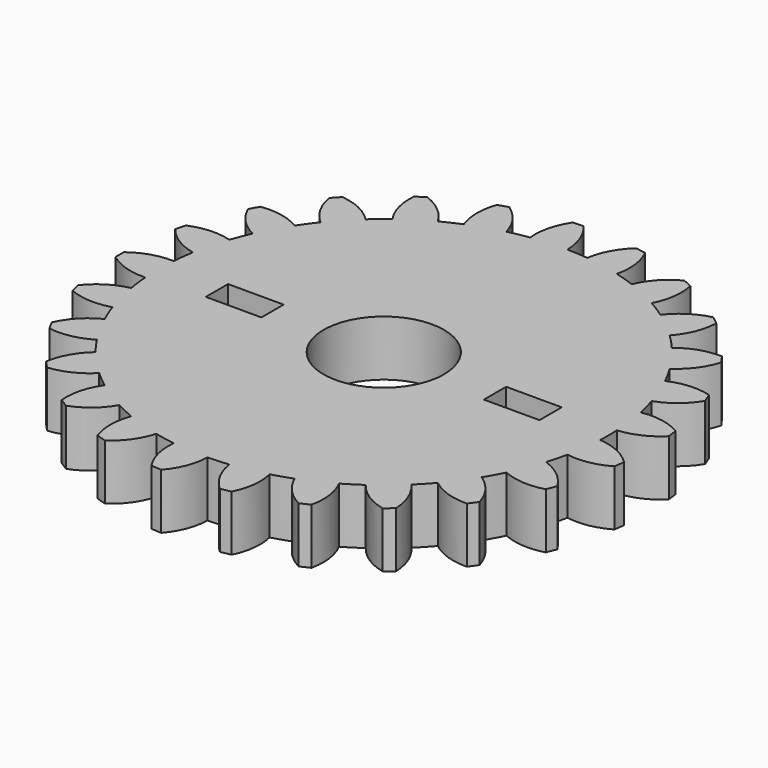
from build123d import *

# Parameters (mm, degrees)
F1_W     = 6
F1_H     = 3
F1_R     = 6.5
F2_DEPTH = 6


# Not quite as in the source:
# - a feature names something its author has since deleted; it is built from what else it names


with BuildPart() as f2:
    # F1 (on Top) → F2 (new body)
    with BuildSketch(Plane.XY):
        with BuildLine():
            ThreePointArc((2.6492001042, 24.1328040773), (1.5244142797, 24.2298711291), (0.3963319999, 24.2745425245))
            ThreePointArc((0.3963319999, 24.2745425245), (-0.0481990645, 26.5171542751), (-1.2314510555, 28.4733828039))
            Line((-1.2314510555, 28.4733828039), (-2.3469204412, 28.4032034187))
            ThreePointArc((-2.3469204412, 28.4032034187), (-3.2756616898, 26.314099538), (-3.4356137115, 24.0334569351))
            ThreePointArc((-3.4356137115, 24.0334569351), (-4.5492019152, 23.8477515871), (-5.6529527401, 23.6104768936))
            ThreePointArc((-5.6529527401, 23.6104768936), (-6.6412329068, 25.672082492), (-8.2738051128, 27.2725897002))
            Line((-8.2738051128, 27.2725897002), (-9.3367770732, 26.9272091737))
            ThreePointArc((-9.3367770732, 26.9272091737), (-9.7168011992, 24.6727697767), (-9.3045552825, 22.4239993048))
            ThreePointArc((-9.3045552825, 22.4239993048), (-10.336975023, 21.9671901071), (-11.3470416693, 21.4628781663))
            ThreePointArc((-11.3470416693, 21.4628781663), (-12.8169736609, 23.2139393506), (-14.796285566, 24.358159484))
            Line((-14.796285566, 24.358159484), (-15.7399696634, 23.7592793451))
            ThreePointArc((-15.7399696634, 23.7592793451), (-15.5473983534, 21.4811591503), (-14.5888574253, 19.4055593285))
            ThreePointArc((-14.5888574253, 19.4055593285), (-15.4752379733, 18.7063492829), (-16.3281542389, 17.9666878688))
            ThreePointArc((-16.3281542389, 17.9666878688), (-18.1873768224, 19.297179025), (-20.3890609801, 19.9132165245))
            Line((-20.3890609801, 19.9132165245), (-21.1541620721, 19.0984666146))
            ThreePointArc((-21.1541620721, 19.0984666146), (-20.4010952897, 16.9398082923), (-18.9564880021, 15.1677966909))
            ThreePointArc((-18.9564880021, 15.1677966909), (-19.6411348079, 14.2701197362), (-20.283308827, 13.3415844957))
            ThreePointArc((-20.283308827, 13.3415844957), (-22.4150002096, 14.1679059711), (-24.7007167071, 14.217052935))
            Line((-24.7007167071, 14.217052935), (-25.2391606782, 13.2376269875))
            ThreePointArc((-25.2391606782, 13.2376269875), (-23.972916379, 11.334066979), (-22.1330127205, 9.9769856039))
            ThreePointArc((-22.1330127205, 9.9769856039), (-22.5729069074, 8.9372460846), (-22.9639885246, 7.8781803018))
            ThreePointArc((-22.9639885246, 7.8781803018), (-25.234206697, 8.1484112791), (-27.4603355605, 7.6275796229))
            Line((-27.4603355605, 7.6275796229), (-27.7382899958, 6.5450185722))
            ThreePointArc((-27.7382899958, 6.5450185722), (-26.038430966, 5.0161645537), (-23.9188388502, 4.1592838187))
            ThreePointArc((-23.9188388502, 4.1592838187), (-24.0863402486, 3.0428123926), (-24.2017563676, 1.9197610656))
            ThreePointArc((-24.2017563676, 1.9197610656), (-26.4678551727, 1.6169219388), (-28.4945205386, 0.5588374309))
            Line((-28.4945205386, 0.5588374309), (-28.4945205386, -0.5588374309))
            ThreePointArc((-28.4945205386, -0.5588374309), (-26.4678551727, -1.6169219388), (-24.2017563676, -1.9197610656))
            ThreePointArc((-24.2017563676, -1.9197610656), (-24.0863402486, -3.0428123926), (-23.9188388502, -4.1592838187))
            ThreePointArc((-23.9188388502, -4.1592838187), (-26.038430966, -5.0161645537), (-27.7382899958, -6.5450185722))
            Line((-27.7382899958, -6.5450185722), (-27.4603355605, -7.6275796229))
            ThreePointArc((-27.4603355605, -7.6275796229), (-25.234206697, -8.1484112791), (-22.9639885246, -7.8781803018))
            ThreePointArc((-22.9639885246, -7.8781803018), (-22.5729069074, -8.9372460846), (-22.1330127205, -9.9769856039))
            ThreePointArc((-22.1330127205, -9.9769856039), (-23.972916379, -11.334066979), (-25.2391606782, -13.2376269875))
            Line((-25.2391606782, -13.2376269875), (-24.7007167071, -14.217052935))
            ThreePointArc((-24.7007167071, -14.217052935), (-22.4150002096, -14.1679059711), (-20.283308827, -13.3415844957))
            ThreePointArc((-20.283308827, -13.3415844957), (-19.6411348079, -14.2701197362), (-18.9564880021, -15.1677966909))
            ThreePointArc((-18.9564880021, -15.1677966909), (-20.4010952897, -16.9398082923), (-21.1541620721, -19.0984666146))
            Line((-21.1541620721, -19.0984666146), (-20.3890609801, -19.9132165245))
            ThreePointArc((-20.3890609801, -19.9132165245), (-18.1873768224, -19.297179025), (-16.3281542389, -17.9666878688))
            ThreePointArc((-16.3281542389, -17.9666878688), (-15.4752379733, -18.7063492829), (-14.5888574253, -19.4055593285))
            ThreePointArc((-14.5888574253, -19.4055593285), (-15.5473983534, -21.4811591503), (-15.7399696634, -23.7592793451))
            Line((-15.7399696634, -23.7592793451), (-14.796285566, -24.358159484))
            ThreePointArc((-14.796285566, -24.358159484), (-12.8169736609, -23.2139393506), (-11.3470416693, -21.4628781663))
            ThreePointArc((-11.3470416693, -21.4628781663), (-10.336975023, -21.9671901071), (-9.3045552825, -22.4239993048))
            ThreePointArc((-9.3045552825, -22.4239993048), (-9.7168011992, -24.6727697767), (-9.3367770732, -26.9272091737))
            Line((-9.3367770732, -26.9272091737), (-8.2738051128, -27.2725897002))
            ThreePointArc((-8.2738051128, -27.2725897002), (-6.6412329068, -25.672082492), (-5.6529527401, -23.6104768936))
            ThreePointArc((-5.6529527401, -23.6104768936), (-4.5492019152, -23.8477515871), (-3.4356137115, -24.0334569351))
            ThreePointArc((-3.4356137115, -24.0334569351), (-3.2756616898, -26.314099538), (-2.3469204412, -28.4032034187))
            Line((-2.3469204412, -28.4032034187), (-1.2314510555, -28.4733828039))
            ThreePointArc((-1.2314510555, -28.4733828039), (-0.0481990645, -26.5171542751), (0.3963319999, -24.2745425245))
            ThreePointArc((0.3963319999, -24.2745425245), (1.5244142797, -24.2298711291), (2.6492001042, -24.1328040773))
            ThreePointArc((2.6492001042, -24.1328040773), (3.3712996907, -26.3020176488), (4.7904018334, -28.0945199331))
            Line((4.7904018334, -28.0945199331), (5.8882796006, -27.8850885483))
            ThreePointArc((5.8882796006, -27.8850885483), (6.5478633024, -25.6960557318), (6.4207137427, -23.413349373))
            ThreePointArc((6.4207137427, -23.413349373), (7.502245919, -23.0895387567), (8.5675549344, -22.7157983851))
            ThreePointArc((8.5675549344, -22.7157983851), (9.8064299128, -24.6372832586), (11.626725543, -26.0205544358))
            Line((11.626725543, -26.0205544358), (12.6380279938, -25.544671625))
            ThreePointArc((12.6380279938, -25.544671625), (12.7324993366, -23.2603795034), (12.0416584273, -21.0810093721))
            ThreePointArc((12.0416584273, -21.0810093721), (13.0086838559, -20.4984057469), (13.9475787787, -19.8714755375))
            ThreePointArc((13.9475787787, -19.8714755375), (15.6253860779, -21.4244977518), (17.7324993267, -22.3116218064))
            Line((17.7324993267, -22.3116218064), (18.5936826087, -21.5991890368))
            ThreePointArc((18.5936826087, -21.5991890368), (18.1171056106, -19.3631680851), (16.9059814268, -17.4240720219))
            ThreePointArc((16.9059814268, -17.4240720219), (17.6977383435, -16.6192825162), (18.4512249528, -15.7785547997))
            ThreePointArc((18.4512249528, -15.7785547997), (20.4625417697, -16.8655322574), (22.724074962, -17.2007679224))
            Line((22.724074962, -17.2007679224), (23.3810277626, -16.2965499651))
            ThreePointArc((23.3810277626, -16.2965499651), (22.3633475091, -14.2492976033), (20.7080394374, -12.6723161452))
            ThreePointArc((20.7080394374, -12.6723161452), (21.2747788433, -11.6959086435), (21.7955128043, -10.6942094344))
            ThreePointArc((21.7955128043, -10.6942094344), (24.0139607061, -11.2468433441), (26.2878133942, -11.0091265299))
            Line((26.2878133942, -11.0091265299), (26.6992569527, -9.9699387246))
            ThreePointArc((26.6992569527, -9.9699387246), (25.2044180369, -8.2400913478), (23.2089351714, -7.1243120397))
            ThreePointArc((23.2089351714, -7.1243120397), (23.5150467452, -6.0376378162), (23.7703084279, -4.9379075597))
            ThreePointArc((23.7703084279, -4.9379075597), (26.0564941741, -4.9214739006), (28.199791831, -4.1257412288))
            Line((28.199791831, -4.1257412288), (28.3398736355, -3.0168795672))
            ThreePointArc((28.3398736355, -3.0168795672), (26.4618022841, -1.713129848), (24.251528152, -1.1286612073))
            ThreePointArc((24.251528152, -1.1286612073), (24.2777777778, 0), (24.251528152, 1.1286612073))
            ThreePointArc((24.251528152, 1.1286612073), (26.4618022841, 1.713129848), (28.3398736355, 3.0168795672))
            Line((28.3398736355, 3.0168795672), (28.199791831, 4.1257412288))
            ThreePointArc((28.199791831, 4.1257412288), (26.0564941741, 4.9214739006), (23.7703084279, 4.9379075597))
            ThreePointArc((23.7703084279, 4.9379075597), (23.5150467452, 6.0376378162), (23.2089351714, 7.1243120397))
            ThreePointArc((23.2089351714, 7.1243120397), (25.2044180369, 8.2400913478), (26.6992569527, 9.9699387246))
            Line((26.6992569527, 9.9699387246), (26.2878133942, 11.0091265299))
            ThreePointArc((26.2878133942, 11.0091265299), (24.0139607061, 11.2468433441), (21.7955128043, 10.6942094344))
            ThreePointArc((21.7955128043, 10.6942094344), (21.2747788433, 11.6959086435), (20.7080394374, 12.6723161452))
            ThreePointArc((20.7080394374, 12.6723161452), (22.3633475091, 14.2492976033), (23.3810277626, 16.2965499651))
            Line((23.3810277626, 16.2965499651), (22.724074962, 17.2007679224))
            ThreePointArc((22.724074962, 17.2007679224), (20.4625417697, 16.8655322574), (18.4512249528, 15.7785547997))
            ThreePointArc((18.4512249528, 15.7785547997), (17.6977383435, 16.6192825162), (16.9059814268, 17.4240720219))
            ThreePointArc((16.9059814268, 17.4240720219), (18.1171056106, 19.3631680851), (18.5936826087, 21.5991890368))
            Line((18.5936826087, 21.5991890368), (17.7324993267, 22.3116218064))
            ThreePointArc((17.7324993267, 22.3116218064), (15.6253860779, 21.4244977518), (13.9475787787, 19.8714755375))
            ThreePointArc((13.9475787787, 19.8714755375), (13.0086838559, 20.4984057469), (12.0416584273, 21.0810093721))
            ThreePointArc((12.0416584273, 21.0810093721), (12.7324993366, 23.2603795034), (12.6380279938, 25.544671625))
            Line((12.6380279938, 25.544671625), (11.626725543, 26.0205544358))
            ThreePointArc((11.626725543, 26.0205544358), (9.8064299128, 24.6372832586), (8.5675549344, 22.7157983851))
            ThreePointArc((8.5675549344, 22.7157983851), (7.502245919, 23.0895387567), (6.4207137427, 23.413349373))
            ThreePointArc((6.4207137427, 23.413349373), (6.5478633024, 25.6960557318), (5.8882796006, 27.8850885483))
            Line((5.8882796006, 27.8850885483), (4.7904018334, 28.0945199331))
            ThreePointArc((4.7904018334, 28.0945199331), (3.3712996907, 26.3020176488), (2.6492001042, 24.1328040773))
        make_face()
        with Locations((-15, 0)):
            Rectangle(F1_W, F1_H, mode=Mode.SUBTRACT)
        Circle(F1_R, mode=Mode.SUBTRACT)
        with Locations((15, 0)):
            Rectangle(F1_W, F1_H, mode=Mode.SUBTRACT)
    extrude(amount=F2_DEPTH)


solid = f2.part
